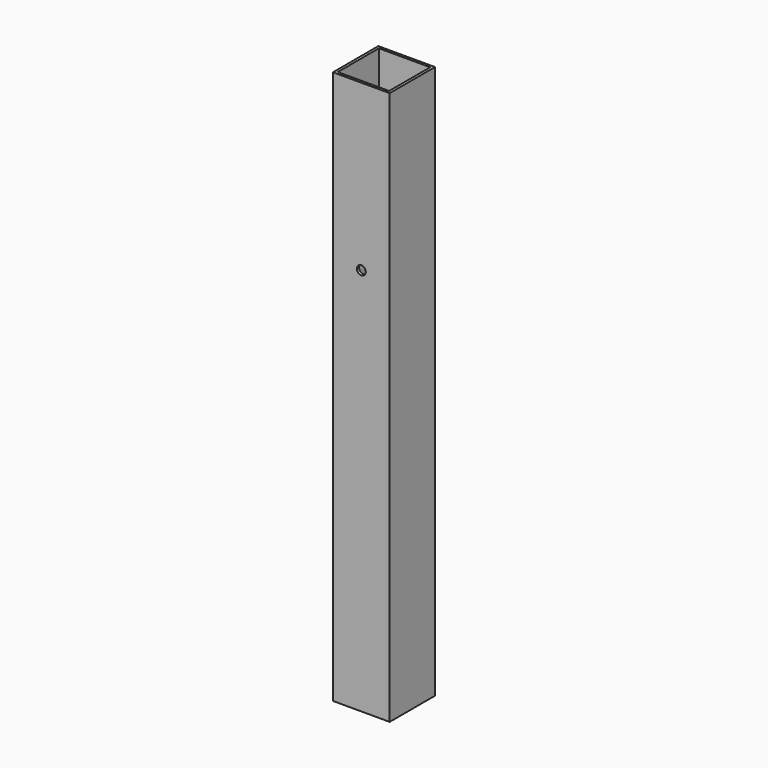
from build123d import *

# Parameters (mm, degrees)
F0_W     = 63.5
F0_H     = 63.5
F0_W_2   = 57.5
F0_H_2   = 57.5
F1_DEPTH = 611
F2_R     = 5
F3_DEPTH = 70


# Not quite as in the source:
# - a pattern or mirror of a feature is missing from the dataset's text; its kind, count and spacing are read off the source's solid


with BuildPart() as f1:
    # F0 (on Top) → F1 (new body)
    with BuildSketch(Plane.XY):
        with Locations((5.5844532326, -0.6013574518)):
            Rectangle(F0_W, F0_H)
        with Locations((5.5844532326, -0.6013574518)):
            Rectangle(F0_W_2, F0_H_2, mode=Mode.SUBTRACT)
    extrude(amount=F1_DEPTH)

    # F1_copies: F1 across plane


with BuildPart() as f1_1:
    add(f1.part)
    add(f1.part.mirror(Plane.XY.offset(310)))

    # F2 (on face) → F3 (cut)
    with BuildSketch(Plane(origin=(0, 31.1486425482, 0), x_dir=(-1, 0, 0), z_dir=(0, 1, 0))):
        with Locations((-5.5844532326, 435)):
            Circle(F2_R)
    extrude(amount=-F3_DEPTH, mode=Mode.SUBTRACT)


solid = f1_1.part
